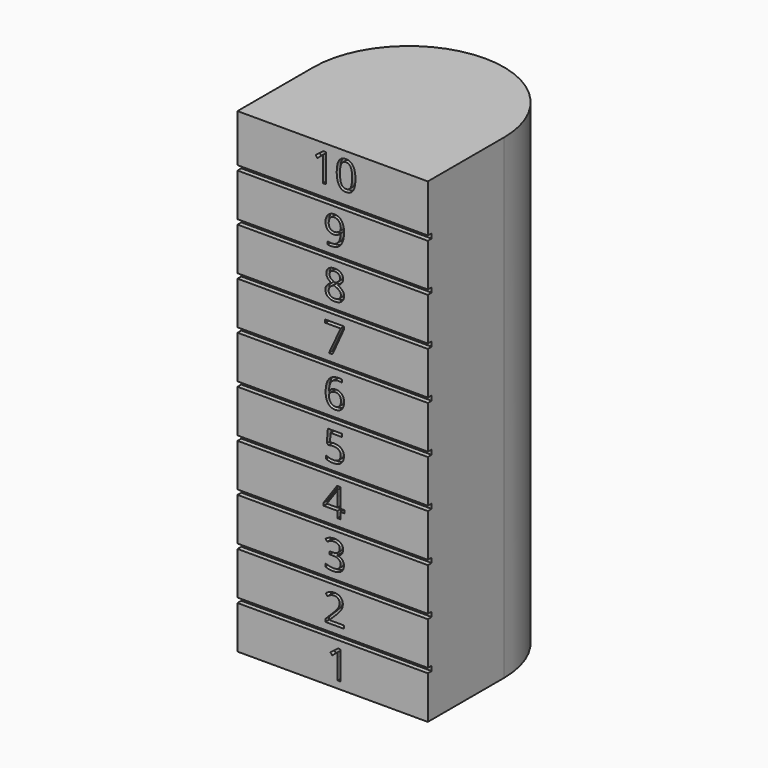
from build123d import *

# Parameters (mm, degrees)
F0_W         = 40
F0_H         = 20
F1_DEPTH     = 100
F2_W         = 45
F2_H         = 1
F2_TEXT_SIZE = 8.3333333333
F3_DEPTH     = 1


# Not quite as in the source:
# - Text() gives the source's letters only with a copy of the font that has no kerning and outlines rounded to 1/6400 em; it was checked with that copy


with BuildPart() as f1:
    # F0 (on Top) → F1 (new body)
    with BuildSketch(Plane.XY):
        with BuildLine():
            ThreePointArc((40, 0), (20, 20), (0, 0))
            Line((0, 0), (40, 0))
        make_face()
        with Locations((20, -10)):
            Rectangle(F0_W, F0_H)
    extrude(amount=F1_DEPTH)

    # F2 (on face) → F3 (cut)
    with BuildSketch(Plane.XZ.offset(20)):
        with Locations((20.5, 9.5)):
            Rectangle(F2_W, F2_H)
        with Locations((20.5, 19.5)):
            Rectangle(F2_W, F2_H)
        with Locations((20.5, 29.5)):
            Rectangle(F2_W, F2_H)
        with Locations((20.5, 39.5)):
            Rectangle(F2_W, F2_H)
        with Locations((20.5, 49.5)):
            Rectangle(F2_W, F2_H)
        with Locations((20.5, 59.5)):
            Rectangle(F2_W, F2_H)
        with Locations((20.5, 69.5)):
            Rectangle(F2_W, F2_H)
        with Locations((20.5, 79.5)):
            Rectangle(F2_W, F2_H)
        with Locations((20.5, 89.5)):
            Rectangle(F2_W, F2_H)
        with Locations((18.775390625, 1.5)):
            Text('1', F2_TEXT_SIZE, font='Open Sans', text_align=(TextAlign.LEFT, TextAlign.BOTTOM))
        with Locations((18.0709635417, 11.5)):
            Text('2', F2_TEXT_SIZE, font='Open Sans', text_align=(TextAlign.LEFT, TextAlign.BOTTOM))
        with Locations((18.091796875, 21.5)):
            Text('3', F2_TEXT_SIZE, font='Open Sans', text_align=(TextAlign.LEFT, TextAlign.BOTTOM))
        with Locations((17.9309895833, 31.5)):
            Text('4', F2_TEXT_SIZE, font='Open Sans', text_align=(TextAlign.LEFT, TextAlign.BOTTOM))
        with Locations((18.0872395833, 41.5)):
            Text('5', F2_TEXT_SIZE, font='Open Sans', text_align=(TextAlign.LEFT, TextAlign.BOTTOM))
        with Locations((18.05078125, 51.5)):
            Text('6', F2_TEXT_SIZE, font='Open Sans', text_align=(TextAlign.LEFT, TextAlign.BOTTOM))
        with Locations((18.0592447917, 61.5)):
            Text('7', F2_TEXT_SIZE, font='Open Sans', text_align=(TextAlign.LEFT, TextAlign.BOTTOM))
        with Locations((18.0631510417, 71.5)):
            Text('8', F2_TEXT_SIZE, font='Open Sans', text_align=(TextAlign.LEFT, TextAlign.BOTTOM))
        with Locations((18.0709635417, 81.5)):
            Text('9', F2_TEXT_SIZE, font='Open Sans', text_align=(TextAlign.LEFT, TextAlign.BOTTOM))
        with Locations((15.6725260417, 92.5)):
            Text('10', F2_TEXT_SIZE, font='Open Sans', text_align=(TextAlign.LEFT, TextAlign.BOTTOM))
    extrude(amount=-F3_DEPTH, mode=Mode.SUBTRACT)


solid = f1.part
